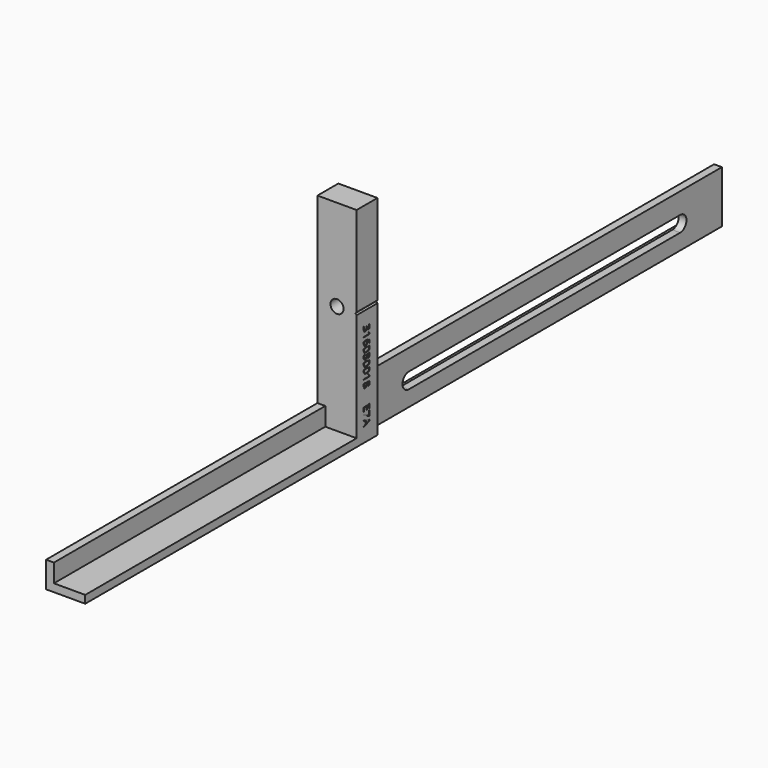
from build123d import *

# Parameters (mm, degrees)
F0_W          = 15
F0_H          = 10
F1_DEPTH      = 80
F3_DEPTH      = 130
F5_DEPTH      = 170
F7_DEPTH      = 5
F9_D          = 5
F10_TEXT_SIZE = 4.1666666667
F11_DEPTH     = 0.2
F13_DEPTH     = 15


# Not quite as in the source:
# - Text() gives the source's letters only with a copy of the font that has no kerning and outlines rounded to 1/6400 em; it was checked with that copy


with BuildPart() as f1:
    # F0 (on Top) → F1 (new body)
    with BuildSketch(Plane.XY):
        Rectangle(F0_W, F0_H)
    extrude(amount=F1_DEPTH)

    # F2 (on face) → F3 (join)
    with BuildSketch(Plane.XZ.offset(5)):
        Polygon((-7.5, 0), (7.5, 0), (7.5, 3), (-4.5, 3), (-4.5, 10), (-7.5, 10), align=None)
    extrude(amount=F3_DEPTH)

    # F4 (on face) → F5 (join)
    with BuildSketch(Plane(origin=(0, 5, 0), x_dir=(-1, 0, 0), z_dir=(0, 1, 0))):
        Polygon((-3.5, 0), (4, 0), (4, 3), (-0.5, 3), (-0.5, 20), (-3.5, 20), align=None)
    extrude(amount=F5_DEPTH)

    # F6 (on face) → F7 (cut)
    with BuildSketch(Plane.YZ.offset(3.5)):
        with BuildLine():
            Line((155, 12), (25, 12))
            ThreePointArc((25, 12), (22, 9), (25, 6))
            Line((25, 6), (155, 6))
            ThreePointArc((155, 6), (158, 9), (155, 12))
        make_face()
    extrude(amount=-F7_DEPTH, mode=Mode.SUBTRACT)

    # F9 (through all)
    with Locations(Plane.XZ.offset(5)):
        with Locations((0, 45)):
            Hole(F9_D / 2)

    # F10 (on face) → F11 (cut)
    with BuildSketch(Plane.YZ.offset(7.5)):
        with Locations(Location((-1.7295359904, 39.458984375), (0, 0, -90))):
            Text('316080018     E7A', F10_TEXT_SIZE, font='Open Sans', text_align=(TextAlign.LEFT, TextAlign.BOTTOM))
    extrude(amount=-F11_DEPTH, mode=Mode.SUBTRACT)

    # F12 (on face) → F13 (cut)
    with BuildSketch(Plane(origin=(0, 5, 0), x_dir=(-1, 0, 0), z_dir=(0, 1, 0))):
        Polygon((-7, 45), (-7.5, 45.5), (-7.5, 44.5), align=None)
    extrude(amount=-F13_DEPTH, mode=Mode.SUBTRACT)


solid = f1.part
